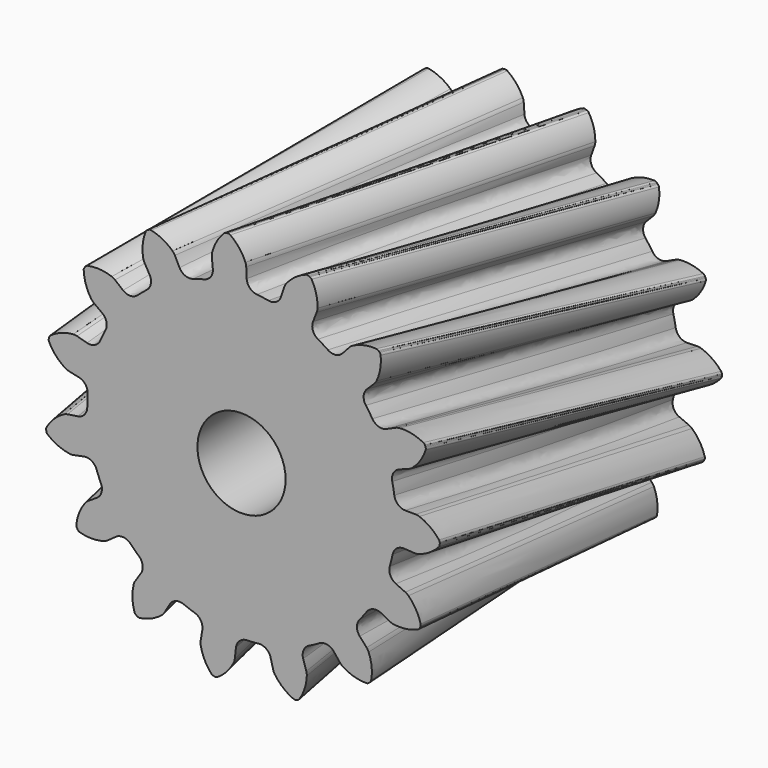
from build123d import *

# Parameters (mm, degrees)
F4_R      = 22.225
F5_DEPTH  = 50.8
F6_COUNT  = 15
F7_R      = 1.6002
F7_2_R    = 1.6002
F7_3_R    = 1.6002
F7_4_R    = 1.6002
F7_5_R    = 1.6002
F7_6_R    = 1.6002
F7_7_R    = 1.6002
F7_8_R    = 1.6002
F7_9_R    = 1.6002
F7_10_R   = 1.6002
F7_11_R   = 1.6002
F7_12_R   = 1.6002
F7_13_R   = 1.6002
F7_14_R   = 1.6002
F7_15_R   = 1.6002
F9_R      = 6.35
F10_DEPTH = 50.8010001


with BuildPart() as f3:
    # F0 (on Front) → F3 section 0
    with BuildSketch(Plane.XZ):
        with BuildLine():
            ThreePointArc((-4.5631032027, 21.7515221114), (-2.1784309438, 22.1179805503), (0.2319130011, 22.2237899864))
            Line((0.2319130011, 22.2237899864), (0.0185531916, 25.1459011236))
            ThreePointArc((0.0185531916, 25.1459011236), (-0.0242941257, 25.4147386606), (-0.1120910603, 25.6724229871))
            ThreePointArc((-0.1120910603, 25.6724229871), (-1.0392535225, 27.1745648018), (-2.3441181542, 28.3634249934))
            ThreePointArc((-2.3441181542, 28.3634249934), (-2.5021196775, 28.4354511085), (-2.675148388, 28.4500561742))
            Line((-2.675148388, 28.4500561742), (-2.8009980611, 28.4390105698))
            Line((-2.8009980611, 28.4390105698), (-2.9265844586, 28.4252918828))
            ThreePointArc((-2.9265844586, 28.4252918828), (-3.0934391639, 28.3772112224), (-3.2343531342, 28.2757445009))
            ThreePointArc((-3.2343531342, 28.2757445009), (-4.2822100404, 26.8551614633), (-4.8985040054, 25.2010024591))
            ThreePointArc((-4.8985040054, 25.2010024591), (-4.9343422284, 24.9311411324), (-4.9239186448, 24.6591101364))
            Line((-4.9239186448, 24.6591101364), (-4.5631032027, 21.7515221114))
        make_face()
    # F2 (on offset) → F3 section 1
    with BuildSketch(Plane.XZ.offset(50.8)):
        with BuildLine():
            ThreePointArc((-12.5397047944, 18.3495620838), (-10.476792476, 19.6007001001), (-8.2904165571, 20.6208539665))
            Line((-8.2904165571, 20.6208539665), (-9.6057788379, 23.2388833737))
            ThreePointArc((-9.6057788379, 23.2388833737), (-9.7482442688, 23.4708599132), (-9.9279695822, 23.675330756))
            ThreePointArc((-9.9279695822, 23.675330756), (-11.3594007898, 24.7083191202), (-13.0198956146, 25.3073326422))
            ThreePointArc((-13.0198956146, 25.3073326422), (-13.193433189, 25.3134115305), (-13.3588799898, 25.2606896309))
            Line((-13.3588799898, 25.2606896309), (-13.4709229572, 25.2023242382))
            Line((-13.4709229572, 25.2023242382), (-13.5816997451, 25.1415899904))
            ThreePointArc((-13.5816997451, 25.1415899904), (-13.7174537202, 25.0333167211), (-13.8088116199, 24.885648252))
            ThreePointArc((-13.8088116199, 24.885648252), (-14.2332715757, 23.1722031818), (-14.1696337106, 21.4081140444))
            ThreePointArc((-14.1696337106, 21.4081140444), (-14.0994724525, 21.1450799939), (-13.9857405618, 20.8977450573))
            Line((-13.9857405618, 20.8977450573), (-12.5397047944, 18.3495620838))
        make_face()
    loft()

    # F4 (on offset) → F5 (join)
    with BuildSketch(Plane.XZ.offset(50.8)):
        Circle(F4_R)
    extrude(amount=-F5_DEPTH)


with BuildPart() as f6_1:
    # F6: instance of F3
    add(f3.part.rotate(Axis((0, -50.8, 0), (0, -1, 0)), 1 * 360 / F6_COUNT))

    # F7#2
    f7_2_edges = [f6_1.edges().sort_by_distance(p)[0] for p in [
        (-12.665438, -25.394088, 18.263003),
        (-16.256265, -25.403004, 15.155345),
    ]]
    fillet(f7_2_edges, radius=F7_2_R)


with BuildPart() as f6_2:
    # F6: instance of F3
    add(f3.part.rotate(Axis((0, -50.8, 0), (0, -1, 0)), 2 * 360 / F6_COUNT))

    # F7#3
    f7_3_edges = [f6_2.edges().sort_by_distance(p)[0] for p in [
        (-18.998686, -25.394088, 11.532586),
        (-21.015071, -25.403004, 7.233078),
    ]]
    fillet(f7_3_edges, radius=F7_3_R)


with BuildPart() as f6_3:
    # F6: instance of F3
    add(f3.part.rotate(Axis((0, -50.8, 0), (0, -1, 0)), 3 * 360 / F6_COUNT))

    # F7#4
    f7_4_edges = [f6_3.edges().sort_by_distance(p)[0] for p in [
        (-22.046889, -25.394088, 2.80808),
        (-22.140181, -25.403004, -1.939854),
    ]]
    fillet(f7_4_edges, radius=F7_4_R)


with BuildPart() as f6_4:
    # F6: instance of F3
    add(f3.part.rotate(Axis((0, -50.8, 0), (0, -1, 0)), 4 * 360 / F6_COUNT))

    # F7#5
    f7_5_edges = [f6_4.edges().sort_by_distance(p)[0] for p in [
        (-21.282984, -25.394088, -6.401969),
        (-19.437052, -25.403004, -10.777367),
    ]]
    fillet(f7_5_edges, radius=F7_5_R)


with BuildPart() as f6_5:
    # F6: instance of F3
    add(f3.part.rotate(Axis((0, -50.8, 0), (0, -1, 0)), 5 * 360 / F6_COUNT))

    # F7#6
    f7_6_edges = [f6_5.edges().sort_by_distance(p)[0] for p in [
        (-16.839058, -25.394088, -14.505059),
        (-13.37308, -25.403004, -17.751376),
    ]]
    fillet(f7_6_edges, radius=F7_6_R)


with BuildPart() as f6_6:
    # F6: instance of F3
    add(f3.part.rotate(Axis((0, -50.8, 0), (0, -1, 0)), 6 * 360 / F6_COUNT))

    # F7#7
    f7_7_edges = [f6_6.edges().sort_by_distance(p)[0] for p in [
        (-9.483506, -25.394088, -20.100093),
        (-4.996782, -25.403004, -21.656011),
    ]]
    fillet(f7_7_edges, radius=F7_7_R)


with BuildPart() as f6_7:
    # F6: instance of F3
    add(f3.part.rotate(Axis((0, -50.8, 0), (0, -1, 0)), 7 * 360 / F6_COUNT))

    # F7#8
    f7_8_edges = [f6_7.edges().sort_by_distance(p)[0] for p in [
        (-0.488169, -25.394088, -22.219638),
        (4.243506, -25.403004, -21.816124),
    ]]
    fillet(f7_8_edges, radius=F7_8_R)


with BuildPart() as f6_8:
    # F6: instance of F3
    add(f3.part.rotate(Axis((0, -50.8, 0), (0, -1, 0)), 8 * 360 / F6_COUNT))

    # F7#9
    f7_9_edges = [f6_8.edges().sort_by_distance(p)[0] for p in [
        (8.591576, -25.394088, -20.497206),
        (12.750053, -25.403004, -18.204032),
    ]]
    fillet(f7_9_edges, radius=F7_9_R)


with BuildPart() as f6_9:
    # F6: instance of F3
    add(f3.part.rotate(Axis((0, -50.8, 0), (0, -1, 0)), 9 * 360 / F6_COUNT))

    # F7#10
    f7_10_edges = [f6_9.edges().sort_by_distance(p)[0] for p in [
        (16.18576, -25.394088, -15.23062),
        (19.052, -25.403004, -11.444297),
    ]]
    fillet(f7_10_edges, radius=F7_10_R)


with BuildPart() as f6_10:
    # F6: instance of F3
    add(f3.part.rotate(Axis((0, -50.8, 0), (0, -1, 0)), 10 * 360 / F6_COUNT))

    # F7#11
    f7_11_edges = [f6_10.edges().sort_by_distance(p)[0] for p in [
        (20.981279, -25.394088, -7.330522),
        (22.059683, -25.403004, -2.705739),
    ]]
    fillet(f7_11_edges, radius=F7_11_R)


with BuildPart() as f6_11:
    # F6: instance of F3
    add(f3.part.rotate(Axis((0, -50.8, 0), (0, -1, 0)), 11 * 360 / F6_COUNT))

    # F7#12
    f7_12_edges = [f6_11.edges().sort_by_distance(p)[0] for p in [
        (22.148944, -25.394088, 1.83709),
        (21.253046, -25.403004, 6.500666),
    ]]
    fillet(f7_12_edges, radius=F7_12_R)


with BuildPart() as f6_12:
    # F6: instance of F3
    add(f3.part.rotate(Axis((0, -50.8, 0), (0, -1, 0)), 12 * 360 / F6_COUNT))

    # F7#13
    f7_13_edges = [f6_12.edges().sort_by_distance(p)[0] for p in [
        (19.486856, -25.394088, 10.687052),
        (16.771565, -25.403004, 14.583046),
    ]]
    fillet(f7_13_edges, radius=F7_13_R)


with BuildPart() as f6_13:
    # F6: instance of F3
    add(f3.part.rotate(Axis((0, -50.8, 0), (0, -1, 0)), 13 * 360 / F6_COUNT))

    # F7#14
    f7_14_edges = [f6_13.edges().sort_by_distance(p)[0] for p in [
        (13.455313, -25.394088, 17.689126),
        (9.390128, -25.403004, 20.143886),
    ]]
    fillet(f7_14_edges, radius=F7_14_R)


with BuildPart() as f6_14:
    # F6: instance of F3
    add(f3.part.rotate(Axis((0, -50.8, 0), (0, -1, 0)), 14 * 360 / F6_COUNT))

    # F7#15
    f7_15_edges = [f6_14.edges().sort_by_distance(p)[0] for p in [
        (5.097224, -25.394088, 21.63259),
        (0.385052, -25.403004, 22.221664),
    ]]
    fillet(f7_15_edges, radius=F7_15_R)


with BuildPart() as f3_1:
    add(f3.part)

    # F7
    f7_edges = [f3_1.edges().sort_by_distance(p)[0] for p in [
        (-4.142221, -25.394088, 21.835582),
        (-8.686603, -25.403004, 20.457115),
    ]]
    fillet(f7_edges, radius=F7_R)


with BuildPart() as f6_14_1:
    add(f6_14.part)

    # F8: union F6_13, F6_12, F6_11, F6_10, F6_9, F6_5, F6_4, F6_3, F6_2, F6_1, F3, F6_6, F6_7, F6_8
    add(f6_13.part)
    add(f6_12.part)
    add(f6_11.part)
    add(f6_10.part)
    add(f6_9.part)
    add(f6_5.part)
    add(f6_4.part)
    add(f6_3.part)
    add(f6_2.part)
    add(f6_1.part)
    add(f3_1.part)
    add(f6_6.part)
    add(f6_7.part)
    add(f6_8.part)

    # F9 (on face) → F10 (cut, through all)
    with BuildSketch(Plane.XZ.offset(50.8)):
        Circle(F9_R)
    extrude(amount=-F10_DEPTH, mode=Mode.SUBTRACT)


solid = f6_14_1.part
